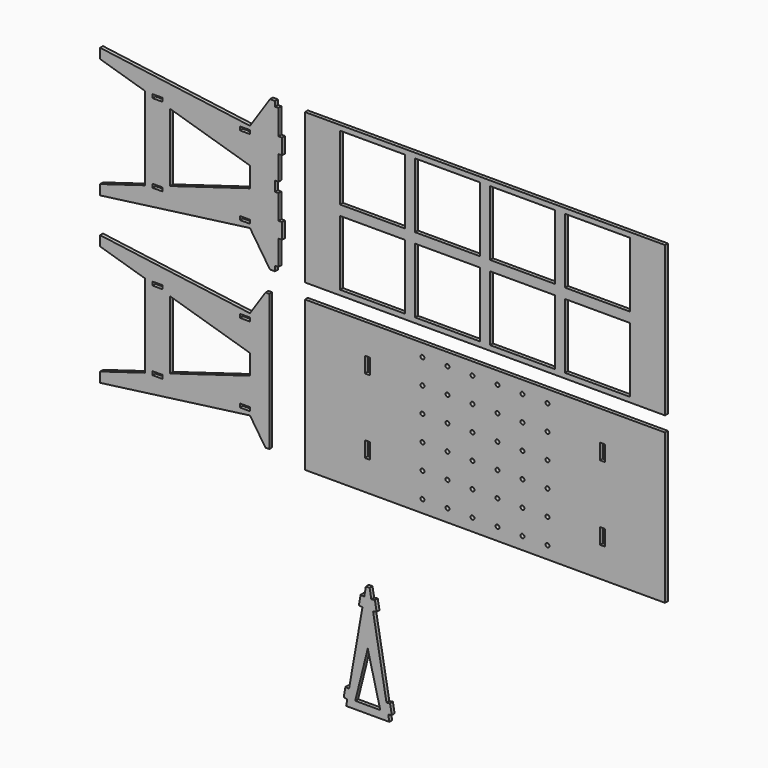
from build123d import *

# Parameters (mm, degrees)
F1_W     = 1828.8
F1_H     = 762
F1_W_2   = 25.0616521179
F1_H_2   = 79.375
F1_R     = 10
F2_DEPTH = 18.288
F1_W_3   = 330.2
F1_H_3   = 330.2
F1_W_4   = 50.8
F1_H_4   = 18.288
F1_W_5   = 17.78
F1_H_5   = 126.9560160066
F1_H_6   = 123.8689839934


# Not quite as in the source:
# - a variable given as a bare number and used for a length is read in inches; the dataset says mm whatever the document's units were
# - a feature names something its author has since deleted; it is built from what else it names


with BuildPart() as f2:
    # F1 (on Front) → F2 (new body)
    with BuildSketch(Plane.XZ):
        with Locations((1473.2, 1524)):
            Rectangle(F1_W, F1_H)
        with Locations((876.130826059, 1335.0435160066)):
            Rectangle(F1_W_2, F1_H_2, mode=Mode.SUBTRACT)
        with Locations((1155.7, 1206.5)):
            Circle(F1_R, mode=Mode.SUBTRACT)
        with Locations((1282.7, 1206.5)):
            Circle(F1_R, mode=Mode.SUBTRACT)
        with Locations((1155.7, 1333.5)):
            Circle(F1_R, mode=Mode.SUBTRACT)
        with Locations((1282.7, 1333.5)):
            Circle(F1_R, mode=Mode.SUBTRACT)
        with Locations((1409.7, 1206.5)):
            Circle(F1_R, mode=Mode.SUBTRACT)
        with Locations((1536.7, 1206.5)):
            Circle(F1_R, mode=Mode.SUBTRACT)
        with Locations((1663.7, 1206.5)):
            Circle(F1_R, mode=Mode.SUBTRACT)
        with Locations((1409.7, 1333.5)):
            Circle(F1_R, mode=Mode.SUBTRACT)
        with Locations((1536.7, 1333.5)):
            Circle(F1_R, mode=Mode.SUBTRACT)
        with Locations((1663.7, 1333.5)):
            Circle(F1_R, mode=Mode.SUBTRACT)
        with Locations((1790.7, 1206.5)):
            Circle(F1_R, mode=Mode.SUBTRACT)
        with Locations((1790.7, 1333.5)):
            Circle(F1_R, mode=Mode.SUBTRACT)
        with Locations((2070.269173941, 1335.0435160066)):
            Rectangle(F1_W_2, F1_H_2, mode=Mode.SUBTRACT)
        with Locations((876.130826059, 1712.9564839934)):
            Rectangle(F1_W_2, F1_H_2, mode=Mode.SUBTRACT)
        with Locations((1155.7, 1460.5)):
            Circle(F1_R, mode=Mode.SUBTRACT)
        with Locations((1282.7, 1460.5)):
            Circle(F1_R, mode=Mode.SUBTRACT)
        with Locations((1155.7, 1587.5)):
            Circle(F1_R, mode=Mode.SUBTRACT)
        with Locations((1282.7, 1587.5)):
            Circle(F1_R, mode=Mode.SUBTRACT)
        with Locations((1155.7, 1714.5)):
            Circle(F1_R, mode=Mode.SUBTRACT)
        with Locations((1282.7, 1714.5)):
            Circle(F1_R, mode=Mode.SUBTRACT)
        with Locations((1409.7, 1460.5)):
            Circle(F1_R, mode=Mode.SUBTRACT)
        with Locations((1409.7, 1587.5)):
            Circle(F1_R, mode=Mode.SUBTRACT)
        with Locations((1536.7, 1460.5)):
            Circle(F1_R, mode=Mode.SUBTRACT)
        with Locations((1663.7, 1460.5)):
            Circle(F1_R, mode=Mode.SUBTRACT)
        with Locations((1536.7, 1587.5)):
            Circle(F1_R, mode=Mode.SUBTRACT)
        with Locations((1663.7, 1587.5)):
            Circle(F1_R, mode=Mode.SUBTRACT)
        with Locations((1409.7, 1714.5)):
            Circle(F1_R, mode=Mode.SUBTRACT)
        with Locations((1536.7, 1714.5)):
            Circle(F1_R, mode=Mode.SUBTRACT)
        with Locations((1663.7, 1714.5)):
            Circle(F1_R, mode=Mode.SUBTRACT)
        with Locations((1155.7, 1841.5)):
            Circle(F1_R, mode=Mode.SUBTRACT)
        with Locations((1282.7, 1841.5)):
            Circle(F1_R, mode=Mode.SUBTRACT)
        with Locations((1409.7, 1841.5)):
            Circle(F1_R, mode=Mode.SUBTRACT)
        with Locations((1536.7, 1841.5)):
            Circle(F1_R, mode=Mode.SUBTRACT)
        with Locations((1663.7, 1841.5)):
            Circle(F1_R, mode=Mode.SUBTRACT)
        with Locations((1790.7, 1460.5)):
            Circle(F1_R, mode=Mode.SUBTRACT)
        with Locations((1790.7, 1587.5)):
            Circle(F1_R, mode=Mode.SUBTRACT)
        with Locations((1790.7, 1714.5)):
            Circle(F1_R, mode=Mode.SUBTRACT)
        with Locations((2070.269173941, 1712.9564839934)):
            Rectangle(F1_W_2, F1_H_2, mode=Mode.SUBTRACT)
        with Locations((1790.7, 1841.5)):
            Circle(F1_R, mode=Mode.SUBTRACT)
    extrude(amount=F2_DEPTH)


with BuildPart() as f2b:
    # F1 (on Front) → F2, piece 2 (new body)
    with BuildSketch(Plane.XZ):
        with Locations((1473.2, 2362.2)):
            Rectangle(F1_W, F1_H)
        with Locations((901.7, 2171.7)):
            Rectangle(F1_W_3, F1_H_3, mode=Mode.SUBTRACT)
        with Locations((901.7, 2552.7)):
            Rectangle(F1_W_3, F1_H_3, mode=Mode.SUBTRACT)
        with Locations((1282.7, 2171.7)):
            Rectangle(F1_W_3, F1_H_3, mode=Mode.SUBTRACT)
        with Locations((1663.7, 2171.7)):
            Rectangle(F1_W_3, F1_H_3, mode=Mode.SUBTRACT)
        with Locations((1282.7, 2552.7)):
            Rectangle(F1_W_3, F1_H_3, mode=Mode.SUBTRACT)
        with Locations((1663.7, 2552.7)):
            Rectangle(F1_W_3, F1_H_3, mode=Mode.SUBTRACT)
        with Locations((2044.7, 2171.7)):
            Rectangle(F1_W_3, F1_H_3, mode=Mode.SUBTRACT)
        with Locations((2044.7, 2552.7)):
            Rectangle(F1_W_3, F1_H_3, mode=Mode.SUBTRACT)
    extrude(amount=F2_DEPTH)


with BuildPart() as f2c:
    # F1 (on Front) → F2, piece 3 (new body)
    with BuildSketch(Plane.XZ):
        Polygon((887.2164165682, 722.2050406681), (868.1664165682, 722.2050406681), (859.5568456234, 673.3777374943), (850.7355181979, 623.3495036413), (782.519362774, 236.4764615814), (773.6980353485, 186.4482277284), (768.1847057076, 155.1805815702), (987.1981274288, 155.1805815702), (981.6847977878, 186.4482277284), (972.8634703624, 236.4764615814), (904.6473149384, 623.3495036413), (895.825987513, 673.3777374943), align=None)
        Polygon((941.1914165682, 193.2805815702), (814.1914165682, 193.2805815702), (877.6914165682, 447.2805815702), align=None, mode=Mode.SUBTRACT)
        Polygon((913.8361517, 676.5534153674), (895.825987513, 673.3777374943), (904.6473149384, 623.3495036413), (922.6574791255, 626.5251815144), align=None)
        Polygon((850.7355181979, 623.3495036413), (859.5568456234, 673.3777374943), (850.5517635298, 674.9655764309), (841.5466814363, 676.5534153674), (832.7253540108, 626.5251815144), align=None)
        Polygon((773.6980353485, 186.4482277284), (782.519362774, 236.4764615814), (773.5142806804, 238.064300518), (764.5091985869, 239.6521394545), (755.6878711614, 189.6239056015), align=None)
        Polygon((990.8736345494, 239.6521394545), (972.8634703624, 236.4764615814), (981.6847977878, 186.4482277284), (999.6949619749, 189.6239056015), align=None)
    extrude(amount=F2_DEPTH)


with BuildPart() as f2d:
    # F1 (on Front) → F2, piece 4 (new body)
    with BuildSketch(Plane.XZ):
        Polygon((406.4, 2511.4689839934), (406.4, 2590.8439839934), (406.4, 2717.8), (406.4, 2743.2), (381, 2743.2), (279.4, 2590.8439839934), (-481.7411823288, 2692.4), (-481.7411823288, 2641.6), (-253.1411823288, 2572.9558292835), (-253.1411823288, 2362.2), (-253.1411823288, 2151.4441707165), (-481.7411823288, 2082.8), (-481.7411823288, 2032), (279.4, 2133.5560160066), (381, 1981.2), (406.4, 1981.2), (406.4, 2006.6), (406.4, 2133.5560160066), (406.4, 2212.9310160066), (406.4, 2336.8), (406.4, 2387.6), align=None)
        with Locations((-189.6411823288, 2161.7500160066)):
            Rectangle(F1_W_4, F1_H_4, mode=Mode.SUBTRACT)
        Polygon((279.4, 2311.3560160066), (-126.1411823288, 2189.5798211145), (-126.1411823288, 2362.2), (-126.1411823288, 2534.8201788855), (279.4, 2413.0439839934), (279.4, 2362.2), align=None, mode=Mode.SUBTRACT)
        with Locations((-189.6411823288, 2562.6499839934)):
            Rectangle(F1_W_4, F1_H_4, mode=Mode.SUBTRACT)
        with Locations((254, 2161.7500160066)):
            Rectangle(F1_W_4, F1_H_4, mode=Mode.SUBTRACT)
        with Locations((254, 2562.6499839934)):
            Rectangle(F1_W_4, F1_H_4, mode=Mode.SUBTRACT)
        Polygon((441.96, 2511.4689839934), (441.96, 2590.8439839934), (424.18, 2590.8439839934), (406.4, 2590.8439839934), (406.4, 2511.4689839934), (424.18, 2511.4689839934), align=None)
        Polygon((441.96, 2212.9310160066), (424.18, 2212.9310160066), (406.4, 2212.9310160066), (406.4, 2133.5560160066), (424.18, 2133.5560160066), (441.96, 2133.5560160066), align=None)
        with Locations((415.29, 2654.3219919967)):
            Rectangle(F1_W_5, F1_H_5)
        with Locations((415.29, 2449.5344919967)):
            Rectangle(F1_W_5, F1_H_6)
        with Locations((415.29, 2274.8655080033)):
            Rectangle(F1_W_5, F1_H_6)
        with Locations((415.29, 2070.0780080033)):
            Rectangle(F1_W_5, F1_H_5)
    extrude(amount=F2_DEPTH)


with BuildPart() as f2e:
    # F1 (on Front) → F2, piece 5 (new body)
    with BuildSketch(Plane.XZ):
        Polygon((-481.7411823288, 1244.6), (-481.7411823288, 1193.8), (279.4, 1295.3560160066), (358.4328318813, 1176.8409825504), (377.4828314781, 1176.8409825504), (377.4828314781, 1871.1590174496), (358.4328318813, 1871.1590174496), (279.4, 1752.6439839934), (-481.7411823288, 1854.2), (-481.7411823288, 1803.4), (-253.1411823288, 1734.7558292835), (-253.1411823288, 1524), (-253.1411823288, 1313.2441707165), align=None)
        with Locations((-189.6411823288, 1323.5500160066)):
            Rectangle(F1_W_4, F1_H_4, mode=Mode.SUBTRACT)
        with Locations((254, 1323.5500160066)):
            Rectangle(F1_W_4, F1_H_4, mode=Mode.SUBTRACT)
        with Locations((-189.6411823288, 1724.4499839934)):
            Rectangle(F1_W_4, F1_H_4, mode=Mode.SUBTRACT)
        Polygon((279.4, 1524), (279.4, 1473.1560160066), (-126.1411823288, 1351.3798211145), (-126.1411823288, 1524), (-126.1411823288, 1696.6201788855), (279.4, 1574.8439839934), align=None, mode=Mode.SUBTRACT)
        with Locations((254, 1724.4499839934)):
            Rectangle(F1_W_4, F1_H_4, mode=Mode.SUBTRACT)
    extrude(amount=F2_DEPTH)


solid = Compound([f2.part, f2b.part, f2c.part, f2d.part, f2e.part])
